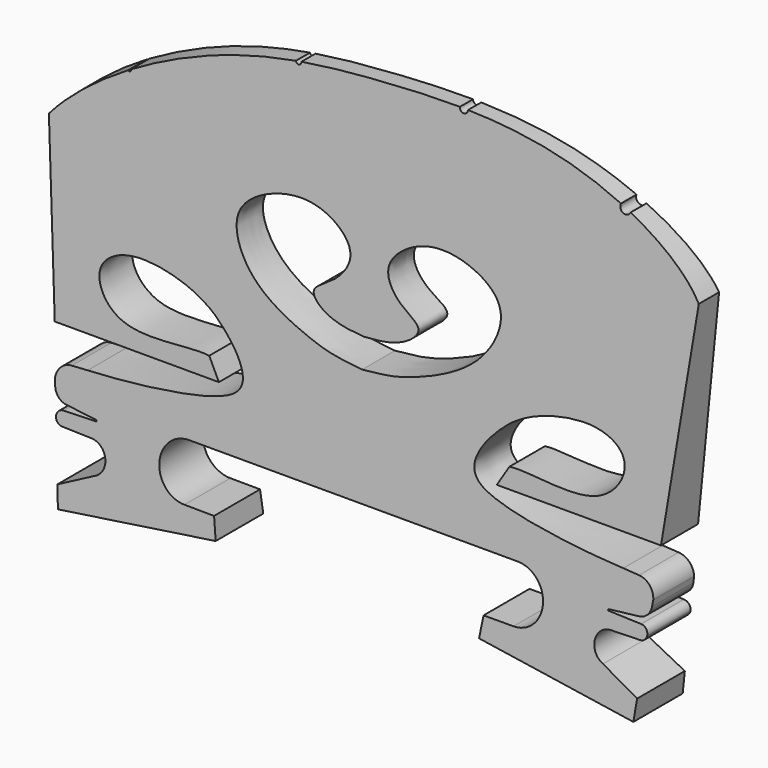
from build123d import *

# Parameters (mm, degrees)
F1_DEPTH     = 4.5
F2_W         = 3.3498070063
F2_H         = 7.5584488809
F2_W_2       = 3.3
F3_DEPTH     = 30
F4_TEXT_SIZE = 3.6633987394
F5_DEPTH     = 0.4


# Not quite as in the source:
# - Text() gives the source's letters only with a copy of the font that has no kerning and outlines rounded to 1/6400 em; it was checked with that copy


with BuildPart() as f1:
    # F0 (on Front) → F1 (new body)
    with BuildSketch(Plane.XZ):
        with BuildLine():
            add(Edge.make_bspline(
                [(-23.5363684416, 23.6552466143), (-22.1809019264, 25.260476146), (-20.2464861976, 26.7563188513), (-18.0861577118, 28.0338079465)],
                knots=[0, 0, 0, 0, 0.1369727751, 0.1369727751, 0.1369727751, 0.1369727751], degree=3))
            Line((-23.5363684416, 23.6552466143), (-22.1226862941, 11.2478661411))
            Line((-22.1226862941, 11.2478661411), (-10.1413011026, 11.2478661411))
            Line((-10.1413011026, 11.2478661411), (-10.9565548074, 12.6261684135))
            add(Edge.make_bspline(
                [(-10.9565548074, 12.6261684135), (-12.4506641968, 12.8114152239), (-17.5784573788, 11.593366016), (-19.9542721652, 15.5722727054), (-16.9274393882, 17.4706918876), (-12.0661208387, 16.3349092226), (-9.9290292696, 14.597388434), (-8.3579108066, 12.6419633785), (-8.3347769443, 9.808542041), (-17.9377850145, 9.0874703601), (-19.545920327, 9.0387157187)],
                knots=[0, 0, 0, 0, 0.1580093991, 0.2698140689, 0.3715152315, 0.5099826839, 0.6153121531, 0.7112759384, 0.7964222327, 1, 1, 1, 1], degree=3))
            Line((-19.545920327, 9.0387157187), (-20.7062717527, 8.9688422158))
            ThreePointArc((-20.7062717527, 8.9688422158), (-21.4957271459, 8.6062784025), (-21.8336324124, 7.8059582369))
            Line((-21.8336324124, 7.8059582369), (-21.7818409617, 7.3668043929))
            ThreePointArc((-21.7818409617, 7.3668043929), (-21.4931945785, 6.7741946047), (-20.8984533479, 6.4899658866))
            Line((-20.8984533479, 6.4899658866), (-18.7077316523, 6.2481180034))
            ThreePointArc((-18.7077316523, 6.2481180034), (-18.6632562021, 6.196469421), (-18.7116228626, 6.1484453865))
            Line((-18.7116228626, 6.1484453865), (-21.0796462954, 6.0728536862))
            ThreePointArc((-21.0796462954, 6.0728536862), (-21.4528495096, 5.9055988754), (-21.5763725918, 5.5157311299))
            Line((-21.5763725918, 5.5157311299), (-21.5706603362, 5.4660585002))
            ThreePointArc((-21.5706603362, 5.4660585002), (-21.3986794627, 5.1939304371), (-21.0964645838, 5.0830373776))
            Line((-21.0964645838, 5.0830373776), (-18.9640834262, 5.0320074941))
            ThreePointArc((-18.9640834262, 5.0320074941), (-17.8633354114, 4.092801096), (-18.5576565569, 2.8232842598))
            Line((-18.5576565569, 2.8232842598), (-21.1583454526, 1.4914511856))
            Line((-21.1583454526, 1.4914511856), (-20.9984287212, 0))
            Line((-20.9984287212, 0), (-9.6103459307, 1.600490661))
            Line((-9.6103459307, 1.600490661), (-9.8450887185, 3.0820087418))
            Line((-9.8450887185, 3.0820087418), (-12.0103669021, 3.0932325061))
            ThreePointArc((-12.0103669021, 3.0932325061), (-13.9999932829, 5.0983891062), (-12, 7.0932056377))
            Line((-12, 7.0932056377), (0, 7.0932056377))
            Line((0, 7.0932056377), (12, 7.0932056377))
            ThreePointArc((12, 7.0932056377), (13.9999969278, 5.0967111581), (12.0070110301, 3.0932179264))
            Line((12.0070110301, 3.0932179264), (9.8222481397, 3.0855591602))
            Line((9.8222481397, 3.0855591602), (9.6134884883, 1.6001570571))
            Line((9.6134884883, 1.6001570571), (21.0015712788, -0.000333604))
            Line((21.0015712788, -0.000333604), (21.1583454526, 1.4914511856))
            Line((21.1583454526, 1.4914511856), (18.5576565569, 2.8232842598))
            ThreePointArc((18.5576565569, 2.8232842598), (17.8633354114, 4.092801096), (18.9640834262, 5.0320074941))
            Line((18.9640834262, 5.0320074941), (21.0964645838, 5.0830373776))
            ThreePointArc((21.0964645838, 5.0830373776), (21.3986794627, 5.1939304371), (21.5706603362, 5.4660585002))
            Line((21.5706603362, 5.4660585002), (21.5763725918, 5.5157311299))
            ThreePointArc((21.5763725918, 5.5157311299), (21.4528495096, 5.9055988754), (21.0796462954, 6.0728536862))
            Line((21.0796462954, 6.0728536862), (18.7116228626, 6.1484453865))
            ThreePointArc((18.7116228626, 6.1484453865), (18.6632562021, 6.196469421), (18.7077316523, 6.2481180034))
            Line((18.7077316523, 6.2481180034), (20.8984533479, 6.4899658866))
            ThreePointArc((20.8984533479, 6.4899658866), (21.4931945785, 6.7741946047), (21.7818409617, 7.3668043929))
            Line((21.7818409617, 7.3668043929), (21.8336324124, 7.8059582369))
            ThreePointArc((21.8336324124, 7.8059582369), (21.4957271459, 8.6062784025), (20.7062717527, 8.9688422158))
            Line((20.7062717527, 8.9688422158), (19.545920327, 9.0387157187))
            add(Edge.make_bspline(
                [(10.9565548074, 12.6261684135), (12.4506641968, 12.8114152239), (17.5784573788, 11.593366016), (19.9542721652, 15.5722727054), (16.9274393882, 17.4706918876), (12.0661208387, 16.3349092226), (9.9290292696, 14.597388434), (8.3579108066, 12.6419633785), (8.3347769443, 9.808542041), (17.9377850145, 9.0874703601), (19.545920327, 9.0387157187)],
                knots=[0, 0, 0, 0, 0.1580093991, 0.2698140689, 0.3715152315, 0.5099826839, 0.6153121531, 0.7112759384, 0.7964222327, 1, 1, 1, 1], degree=3))
            Line((10.9565548074, 12.6261684135), (10.1413011026, 11.2478661411))
            Line((10.1413011026, 11.2478661411), (22.1226862941, 11.2478661411))
            Line((22.1226862941, 11.2478661411), (23.6598201241, 26.6479611198))
            add(Edge.make_bspline(
                [(18.3638422533, 30.6360920918), (20.7414594365, 29.525659305), (22.7102987642, 28.1182143601), (23.6598201241, 26.6479611198)],
                knots=[0.851348028, 0.851348028, 0.851348028, 0.851348028, 1, 1, 1, 1], degree=3))
            ThreePointArc((18.3638422533, 30.6360920918), (17.8368362551, 30.4370722143), (17.6334494669, 30.962408343))
            add(Edge.make_bspline(
                [(6.299949222, 33.1952163198), (8.8406655698, 33.1403760478), (12.7089048862, 32.7453965852), (16.4623871501, 31.4626658371), (17.6334494669, 30.962408343)],
                knots=[0.6233705909, 0.6233705909, 0.6233705909, 0.6233705909, 0.7654288362, 0.8363726665, 0.8363726665, 0.8363726665, 0.8363726665], degree=3))
            ThreePointArc((6.299949222, 33.1952163198), (5.9954147324, 32.9007708022), (5.7000222178, 33.2043868105))
            add(Edge.make_bspline(
                [(-5.8025069017, 32.3939596743), (-3.9020740666, 32.693179971), (-0.2174126257, 33.0225352164), (3.7593850718, 33.2220932827), (5.7000222178, 33.2043868105)],
                knots=[0.3860705679, 0.3860705679, 0.3860705679, 0.3860705679, 0.5033806167, 0.6121750006, 0.6121750006, 0.6121750006, 0.6121750006], degree=3))
            ThreePointArc((-5.8025069017, 32.3939596743), (-5.8006277105, 32.3782258626), (-5.8, 32.3623926643))
            ThreePointArc((-5.8, 32.3623926643), (-5.9836956637, 32.1630583506), (-6.1973416862, 32.3298925274))
            add(Edge.make_bspline(
                [(-17.9136809927, 28.135058526), (-16.0575985182, 29.2167312118), (-11.9733823838, 31.0824601466), (-8.1447664633, 32.0043795548), (-6.1973416862, 32.3298925274)],
                knots=[0.1406080449, 0.1406080449, 0.1406080449, 0.1406080449, 0.2576542794, 0.3779435559, 0.3779435559, 0.3779435559, 0.3779435559], degree=3))
            ThreePointArc((-17.9136809927, 28.135058526), (-17.903480829, 28.1107249593), (-17.9, 28.0845706167))
            ThreePointArc((-17.9, 28.0845706167), (-17.9736919327, 27.9880932329), (-18.0861577118, 28.0338079465))
        make_face()
        with BuildLine():
            add(Edge.make_bspline(
                [(0, 15.1957957089), (2.0903856573, 15.3791947525), (3.6702107386, 15.777829192), (8.5046642167, 17.7997724532), (10.4334916547, 22.0389484407), (7.17305578, 24.1425953549), (3.6327140381, 24.4256207343), (0.659762582, 22.1035580099), (2.2932652276, 19.8200812112), (4.4103600725, 18.9883550435), (2.6764111625, 17.4313099969), (0.8823938701, 17.2681713059), (0, 17.2159889728)],
                knots=[0, 0, 0, 0, 0.1171327199, 0.2437561037, 0.355967299, 0.4582118124, 0.5680705646, 0.6675254018, 0.7551120606, 0.8310829496, 0.9031037961, 1, 1, 1, 1], degree=3))
            add(Edge.make_bspline(
                [(0, 15.1957957089), (-2.0903856573, 15.3791947525), (-3.6702107386, 15.777829192), (-8.5046642167, 17.7997724532), (-10.4334916547, 22.0389484407), (-7.17305578, 24.1425953549), (-3.6327140381, 24.4256207343), (-0.659762582, 22.1035580099), (-2.2932652276, 19.8200812112), (-4.4103600725, 18.9883550435), (-2.6764111625, 17.4313099969), (-0.8823938701, 17.2681713059), (0, 17.2159889728)],
                knots=[0, 0, 0, 0, 0.1171327199, 0.2437561037, 0.355967299, 0.4582118124, 0.5680705646, 0.6675254018, 0.7551120606, 0.8310829496, 0.9031037961, 1, 1, 1, 1], degree=3))
        make_face(mode=Mode.SUBTRACT)
    extrude(amount=F1_DEPTH)

    # F2 (on Right) → F3 (cut, symmetric)
    with BuildSketch(Plane.YZ):
        Polygon((-4.5, 0), (-4.5, 33.213060528), (-7.8498070063, 33.213060528), (-9.0029938146, 0), align=None)
        Polygon((-4.5, 0), (-1.2, 33.213060528), (-4.5, 33.213060528), align=None)
        with Locations((-6.1749035031, 36.9922849685)):
            Rectangle(F2_W, F2_H)
        with Locations((-2.85, 36.9922849685)):
            Rectangle(F2_W_2, F2_H)
    extrude(amount=F3_DEPTH, both=True, mode=Mode.SUBTRACT)

    # F4 (on face) → F5 (cut)
    with BuildSketch(Plane(origin=(0, 0, 0), x_dir=(-1, 0, 0), z_dir=(0, 1, 0))):
        with Locations((-6.1517595313, 10.8835203573)):
            Text('justnth', F4_TEXT_SIZE, font='Open Sans', text_align=(TextAlign.LEFT, TextAlign.BOTTOM))
    extrude(amount=-F5_DEPTH, mode=Mode.SUBTRACT)


solid = f1.part
